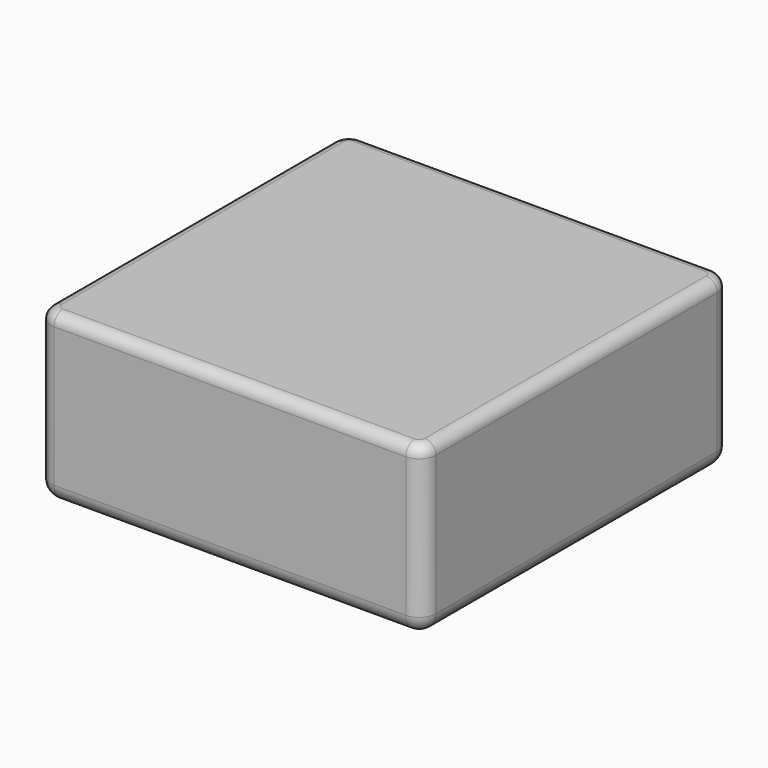
from build123d import *

# Parameters (mm, degrees)
F0_W     = 175.26
F0_H     = 175.26
F1_DEPTH = 71.12
F2_R     = 7.62
F3_T     = -2.54
F5_DEPTH = 5.08
F6_R     = 5.07999


# Not quite as in the source:
# - a fillet or chamfer is up to 0.001 mm smaller than in the source, because OpenCascade refuses the exact size


with BuildPart() as f1:
    # F0 (on Top) → F1 (new body)
    with BuildSketch(Plane.XY):
        Rectangle(F0_W, F0_H)
    extrude(amount=F1_DEPTH)

    # F2
    f2_edges = [f1.edges().sort_by_distance(p)[0] for p in [
        (-87.63, 87.63, 35.56),
        (87.63, 87.63, 35.56),
        (-87.63, -87.63, 35.56),
        (87.63, -87.63, 35.56),
        (-87.63, 0, 0),
        (0, -87.63, 0),
        (0, 87.63, 0),
        (87.63, 0, 0),
    ]]
    fillet(f2_edges, radius=F2_R)

    # F3
    f3_openings = [f1.faces().sort_by_distance(p)[0] for p in [
        (0, 0, 71.12),
    ]]
    offset(amount=F3_T, openings=f3_openings)


with BuildPart() as f5:
    # F4 (on face) → F5 (new body)
    with BuildSketch(Plane.XY.offset(71.12)):
        with BuildLine():
            Line((80.01, 87.63), (-80.01, 87.63))
            ThreePointArc((-80.01, 87.63), (-85.3981536726, 85.3981536726), (-87.63, 80.01))
            Line((-87.63, 80.01), (-87.63, -80.01))
            ThreePointArc((-87.63, -80.01), (-85.3981536726, -85.3981536726), (-80.01, -87.63))
            Line((-80.01, -87.63), (80.01, -87.63))
            ThreePointArc((80.01, -87.63), (85.3981536726, -85.3981536726), (87.63, -80.01))
            Line((87.63, -80.01), (87.63, 80.01))
            ThreePointArc((87.63, 80.01), (85.3981536726, 85.3981536726), (80.01, 87.63))
        make_face()
    extrude(amount=F5_DEPTH)

    # F6 (radius 5.08 in the source; OpenCascade refuses exactly that, so slightly less here)
    f6_edges = [f5.edges().sort_by_distance(p)[0] for p in [
        (87.63, 0, 76.2),
    ]]
    fillet(f6_edges, radius=F6_R)


solid = Compound([f1.part, f5.part])
